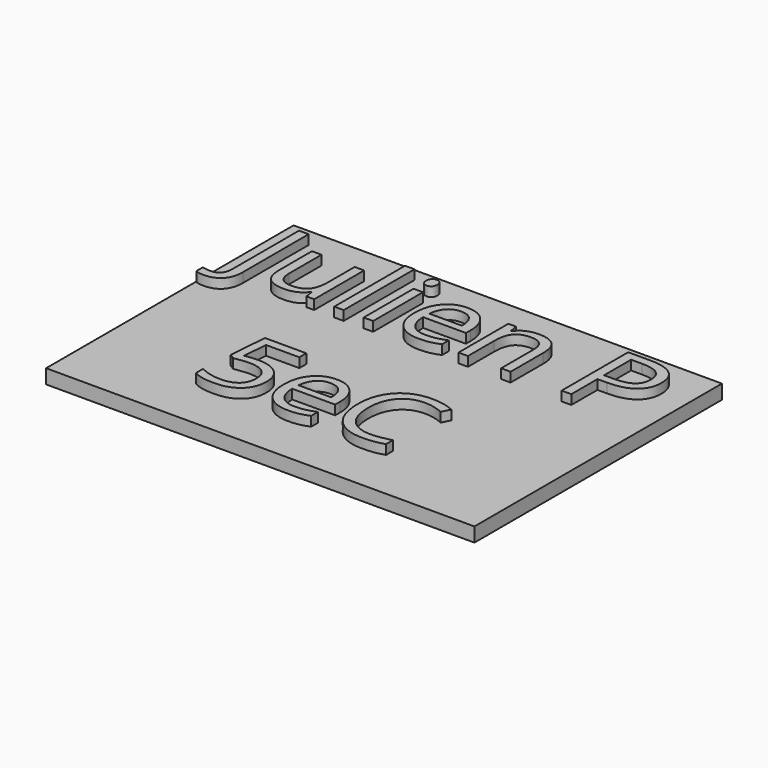
from build123d import *

# Parameters (mm, degrees)
F0_W         = 90
F0_H         = 65
F1_DEPTH     = 3
F2_TEXT_SIZE = 24.4654842868
F3_DEPTH     = 2


# Not quite as in the source:
# - Text() gives the source's letters only with a copy of the font that has no kerning and outlines rounded to 1/6400 em; it was checked with that copy


with BuildPart() as f1:
    # F0 (on Top) → F1 (new body)
    with BuildSketch(Plane.XY):
        with Locations((45, 32.5)):
            Rectangle(F0_W, F0_H)
    extrude(amount=F1_DEPTH)

    # F2 (on face) → F3 (join)
    with BuildSketch(Plane.XY.offset(3)):
        with Locations((2, 43.6197599993)):
            Text('Julien P', F2_TEXT_SIZE, font='Open Sans', text_align=(TextAlign.LEFT, TextAlign.BOTTOM))
        with Locations((21.0716095479, 10.3467013692)):
            Text('5eC', F2_TEXT_SIZE, font='Open Sans', text_align=(TextAlign.LEFT, TextAlign.BOTTOM))
    extrude(amount=F3_DEPTH)


solid = f1.part
